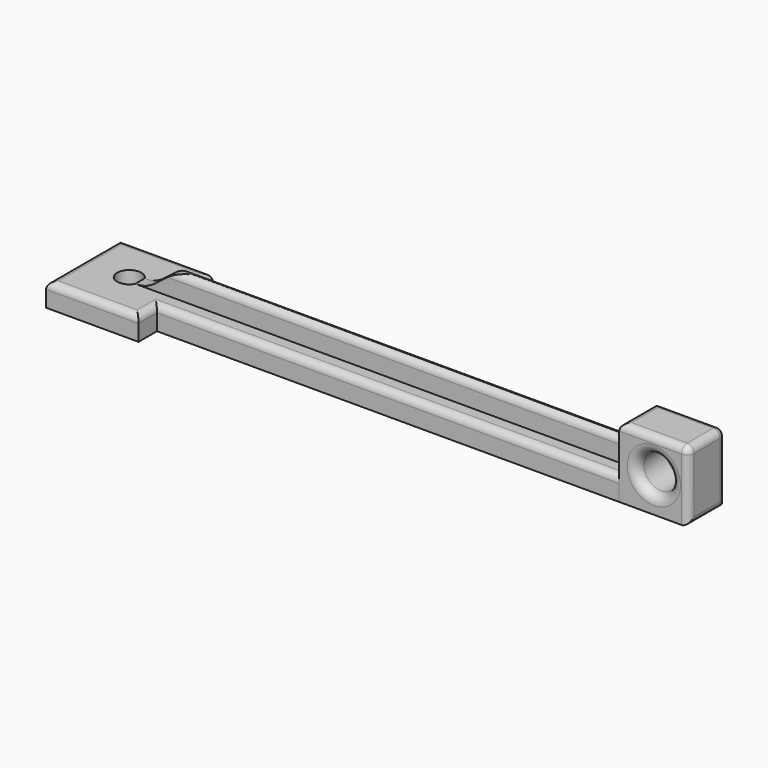
from build123d import *

# Parameters (mm, degrees)
F0_W          = 100
F0_H          = 3.75
F1_DEPTH      = 5
F0_H_2        = 2.5
F2_DEPTH      = 10
F3_DEPTH      = 15
F4_R          = 3.75
F5_DEPTH      = 30.025
F6_R          = 1.5
F7_T1_DEPTH   = 103.75
F7_T3_DEPTH   = 27.5
F7_T5_DEPTH   = 8.75
F7_T7_DEPTH   = 8.75
F7_T9_DEPTH   = 27.5
F7_T15_DEPTH  = 12.5
F7_T19_DEPTH  = 107.5
F7_T26_DEPTH  = 107.5
F7_T30_DEPTH  = 12.5
F7_2_T1_DEPTH = 117.5
F9_DEPTH      = 25
F9_FACE_W     = 2.3082731641
F9_FACE_H     = 2.5
F10_DEPTH     = 25
F11_R         = 2


# Not quite as in the source:
# - a fillet or chamfer that OpenCascade refuses, or shapes differently, is made with other operations: its cross-section is extruded or revolved along the edge and cut away or added
# - a feature names something its author has since deleted; it is built from what else it names


with BuildPart() as f1:
    # F0 (on Top) → F1 (new body)
    with BuildSketch(Plane.XY):
        with BuildLine():
            Line((10, 10), (-10, 10))
            Line((-10, 10), (-10, -10))
            Line((-10, -10), (10, -10))
            Line((10, -10), (10, -5))
            Line((10, -5), (10, -1.25))
            Line((10, -1.25), (2.3082731641, -1.25))
            ThreePointArc((2.3082731641, -1.25), (-2.625, 0), (2.3082731641, 1.25))
            Line((2.3082731641, 1.25), (10, 1.25))
            Line((10, 1.25), (10, 5))
            Line((10, 5), (10, 10))
        make_face()
        with Locations((60, 3.125)):
            Rectangle(F0_W, F0_H)
        with Locations((60, -3.125)):
            Rectangle(F0_W, F0_H)
    extrude(amount=F1_DEPTH)

    # F7: fillet of radius 1.5 on 7 edges, made by hand

    # F7_s2 → F7_t1 (cut)
    with BuildSketch(Plane.YZ.offset(10)):
        with BuildLine():
            ThreePointArc((-5, 3.5), (-4.5606601718, 4.5606601718), (-3.5, 5))
            Line((-3.5, 5), (-5, 5))
            Line((-5, 5), (-5, 3.5))
        make_face()
        with BuildLine():
            ThreePointArc((5, 3.5), (4.5606601718, 4.5606601718), (3.5, 5))
            Line((3.5, 5), (5, 5))
            Line((5, 5), (5, 3.5))
        make_face()
    extrude(amount=F7_T1_DEPTH, mode=Mode.SUBTRACT)

    # F7_s4 → F7_t3 (cut)
    with BuildSketch(Plane.YZ.offset(-13.75)):
        with BuildLine():
            ThreePointArc((10, 3.5), (9.5606601718, 4.5606601718), (8.5, 5))
            Line((8.5, 5), (10, 5))
            Line((10, 5), (10, 3.5))
        make_face()
        with BuildLine():
            ThreePointArc((-10, 3.5), (-9.5606601718, 4.5606601718), (-8.5, 5))
            Line((-8.5, 5), (-10, 5))
            Line((-10, 5), (-10, 3.5))
        make_face()
    extrude(amount=F7_T3_DEPTH, mode=Mode.SUBTRACT)

    # F7_s6 → F7_t5 (cut)
    with BuildSketch(Plane.XZ.offset(-13.75)):
        with BuildLine():
            ThreePointArc((10, 3.5), (9.5606601718, 4.5606601718), (8.5, 5))
            Line((8.5, 5), (10, 5))
            Line((10, 5), (10, 3.5))
        make_face()
    extrude(amount=F7_T5_DEPTH, mode=Mode.SUBTRACT)

    # F7_s8 → F7_t7 (cut)
    with BuildSketch(Plane.XZ.offset(5)):
        with BuildLine():
            ThreePointArc((10, 3.5), (9.5606601718, 4.5606601718), (8.5, 5))
            Line((8.5, 5), (10, 5))
            Line((10, 5), (10, 3.5))
        make_face()
    extrude(amount=F7_T7_DEPTH, mode=Mode.SUBTRACT)

    # F7_s10 → F7_t9 (cut)
    with BuildSketch(Plane.XZ.offset(-13.75)):
        with BuildLine():
            ThreePointArc((-10, 3.5), (-9.5606601718, 4.5606601718), (-8.5, 5))
            Line((-8.5, 5), (-10, 5))
            Line((-10, 5), (-10, 3.5))
        make_face()
    extrude(amount=F7_T9_DEPTH, mode=Mode.SUBTRACT)


with BuildPart() as f2:
    # F0 (on Top) → F2 (new body)
    with BuildSketch(Plane.XY):
        with BuildLine():
            ThreePointArc((2.625, 0), (2.5445866124, 0.6447510932), (2.3082731641, 1.25))
            Line((2.3082731641, 1.25), (0, 1.25))
            Line((0, 1.25), (0, -1.25))
            Line((0, -1.25), (2.3082731641, -1.25))
            ThreePointArc((2.3082731641, -1.25), (2.5445866124, -0.6447510932), (2.625, 0))
        make_face()
        with BuildLine():
            Line((10, -1.25), (10, 1.25))
            Line((10, 1.25), (2.3082731641, 1.25))
            ThreePointArc((2.3082731641, 1.25), (2.5445866124, 0.6447510932), (2.625, 0))
            ThreePointArc((2.625, 0), (2.5445866124, -0.6447510932), (2.3082731641, -1.25))
            Line((2.3082731641, -1.25), (10, -1.25))
        make_face()
        with Locations((60, 0)):
            Rectangle(F0_W, F0_H_2)
    extrude(amount=F2_DEPTH)

    # F7#2: fillet of radius 1.5 on 2 edges, made by hand

    # F7_2_s2 → F7_2_t1 (cut)
    with BuildSketch(Plane.YZ.offset(-3.75)):
        with BuildLine():
            ThreePointArc((-1.25, 8.5), (-0.8106601718, 9.5606601718), (0.25, 10))
            Line((0.25, 10), (-1.25, 10))
            Line((-1.25, 10), (-1.25, 8.5))
        make_face()
        with BuildLine():
            ThreePointArc((1.25, 8.5), (0.8106601718, 9.5606601718), (-0.25, 10))
            Line((-0.25, 10), (1.25, 10))
            Line((1.25, 10), (1.25, 8.5))
        make_face()
    extrude(amount=F7_2_T1_DEPTH, mode=Mode.SUBTRACT)

    # F8 (on face) → F9 (cut)
    with BuildSketch(Plane.XZ.offset(1.25)):
        with BuildLine():
            Line((0, 5), (2.3082731641, 5))
            add(Edge.make_bspline(
                [(2.3082731641, 5), (5.7885707555, 5), (7.0454086994, 7.0322147924), (9.2201348345, 8.5)],
                knots=[0, 0, 0, 0, 8.3278889996, 8.3278889996, 8.3278889996, 8.3278889996], degree=3))
            Line((9.2201348345, 8.5), (0, 8.5))
            Line((0, 8.5), (0, 5))
        make_face()
        with BuildLine():
            Line((0, 8.5), (9.2201348345, 8.5))
            add(Edge.make_bspline(
                [(9.2201348345, 8.5), (10.4494255604, 9.3296836618), (11.9720012822, 9.9790199458), (14.3552316788, 9.9790199458)],
                knots=[8.3278889996, 8.3278889996, 8.3278889996, 8.3278889996, 13.0353308004, 13.0353308004, 13.0353308004, 13.0353308004], degree=3))
            Line((14.3552316788, 9.9790199458), (0, 9.9790199458))
            Line((0, 9.9790199458), (0, 8.5))
        make_face()
    extrude(amount=-F9_DEPTH, mode=Mode.SUBTRACT)

    # F0 (on Top) + F9_face (on face) → F10 (cut)
    with BuildSketch(Plane.XY):
        with BuildLine():
            Line((0, 1.25), (2.3082731641, 1.25))
            ThreePointArc((2.3082731641, 1.25), (-2.625, 0), (2.3082731641, -1.25))
            Line((2.3082731641, -1.25), (0, -1.25))
            Line((0, -1.25), (0, 1.25))
        make_face()
    with BuildSketch(Plane(origin=(1.154136582, 0, 5), x_dir=(1, 0, 0), z_dir=(0, 0, 1))):
        Rectangle(F9_FACE_W, F9_FACE_H)
    extrude(amount=-F10_DEPTH, mode=Mode.SUBTRACT)


with BuildPart() as f3:
    # F0 (on Top) → F3 (new body)
    with BuildSketch(Plane.XY):
        Polygon((125, 5), (110, 5), (110, 1.25), (110, -1.25), (110, -5), (125, -5), align=None)
    extrude(amount=F3_DEPTH)

    # F4 (on face) → F5 (cut)
    with BuildSketch(Plane.XZ.offset(5)):
        with Locations((117.5, 7.5)):
            Circle(F4_R)
    extrude(amount=-F5_DEPTH, mode=Mode.SUBTRACT)

    # F6
    f6_edges = [f3.edges().sort_by_distance(p)[0] for p in [
        (110, 0, 15),
        (125, 0, 15),
        (125, 0, 0),
        (117.5, -5, 15),
        (125, -5, 7.5),
        (117.5, 5, 15),
        (125, 5, 7.5),
    ]]
    fillet(f6_edges, radius=F6_R)

    # F11
    f11_edges = [f3.edges().sort_by_distance(p)[0] for p in [
        (113.75, -5, 7.5),
        (113.75, 5, 7.5),
    ]]
    fillet(f11_edges, radius=F11_R)


with BuildPart() as f7_tool13:
    # F7_s14 → F7_t15 (new body)
    with BuildSketch(Plane.XZ.offset(13.75)):
        with BuildLine():
            ThreePointArc((10, 3.5), (9.5606601718, 4.5606601718), (8.5, 5))
            Line((8.5, 5), (10, 5))
            Line((10, 5), (10, 3.5))
        make_face()
    extrude(amount=-F7_T15_DEPTH)

    split(bisect_by=Plane.XZ.offset(5), keep=Keep.BOTTOM)


with BuildPart() as f7_tool17:
    # F7_s18 → F7_t19 (new body)
    with BuildSketch(Plane.YZ.offset(6.25)):
        with BuildLine():
            ThreePointArc((-5, 3.5), (-4.5606601718, 4.5606601718), (-3.5, 5))
            Line((-3.5, 5), (-5, 5))
            Line((-5, 5), (-5, 3.5))
        make_face()
    extrude(amount=F7_T19_DEPTH)

    split(bisect_by=Plane.YZ.offset(10), keep=Keep.BOTTOM)


with BuildPart() as f7_tool13_1:
    add(f7_tool13.part)

    # F7_t21: intersect F7_tool17
    add(f7_tool17.part, mode=Mode.INTERSECT)


with BuildPart() as f1_1:
    add(f1.part)

    # F7_t11: cut F7_tool13
    add(f7_tool13_1.part, mode=Mode.SUBTRACT)


with BuildPart() as f7_tool24:
    # F7_s25 → F7_t26 (new body)
    with BuildSketch(Plane.YZ.offset(113.75)):
        with BuildLine():
            ThreePointArc((5, 3.5), (4.5606601718, 4.5606601718), (3.5, 5))
            Line((3.5, 5), (5, 5))
            Line((5, 5), (5, 3.5))
        make_face()
    extrude(amount=-F7_T26_DEPTH)

    split(bisect_by=Plane.YZ.offset(10), keep=Keep.BOTTOM)


with BuildPart() as f7_tool28:
    # F7_s29 → F7_t30 (new body)
    with BuildSketch(Plane.XZ.offset(-1.25)):
        with BuildLine():
            ThreePointArc((10, 3.5), (9.5606601718, 4.5606601718), (8.5, 5))
            Line((8.5, 5), (10, 5))
            Line((10, 5), (10, 3.5))
        make_face()
    extrude(amount=-F7_T30_DEPTH)

    split(bisect_by=Plane.XZ.offset(-5), keep=Keep.TOP)


with BuildPart() as f7_tool24_1:
    add(f7_tool24.part)

    # F7_t32: intersect F7_tool28
    add(f7_tool28.part, mode=Mode.INTERSECT)


with BuildPart() as f1_2:
    add(f1_1.part)

    # F7_t22: cut F7_tool24
    add(f7_tool24_1.part, mode=Mode.SUBTRACT)


solid = Compound([f2.part, f3.part, f1_2.part])
